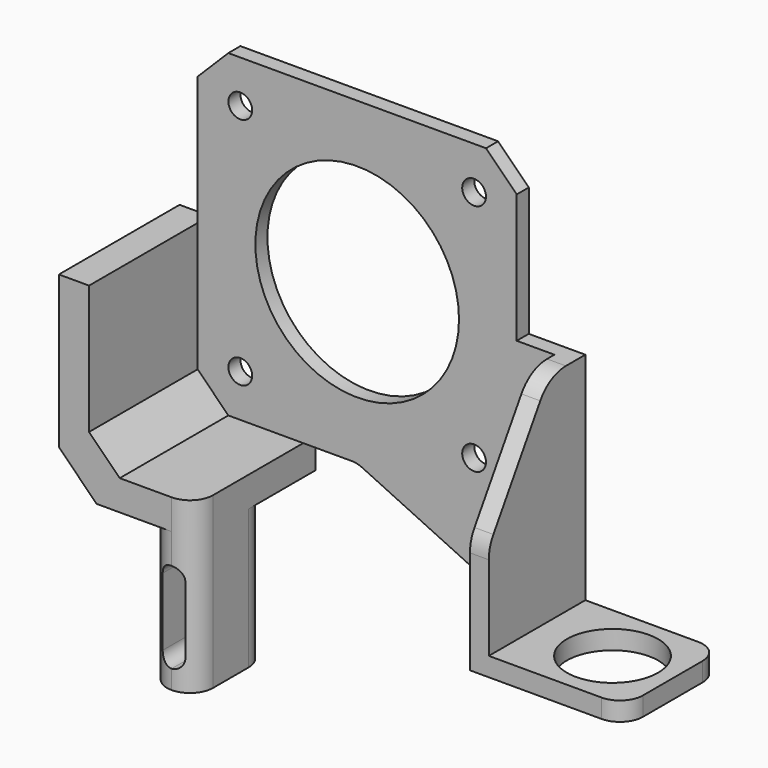
from build123d import *

# Parameters (mm, degrees)
F0_R         = 1.575
F0_R_2       = 13.5
F0_W         = 5
F0_H         = 21.15
F1_DEPTH     = 2
F2_DEPTH     = 20
F3_DEPTH     = 16
F4_R         = 6.05
F5_DEPTH     = 2.5
F6_W         = 6.1
F6_H         = 12
F7_DEPTH     = 18.5
F8_W         = 3
F8_H         = 12
F9_DEPTH     = 12
F10_T1_DEPTH = 2
F10_T3_DEPTH = 26.125
F10_T5_DEPTH = 37.75
F10_T7_DEPTH = 17.75
F10_T9_DEPTH = 5.4173756904
F11_R        = 1.49999
F12_SIZE     = 5
F13_SIZE2    = 16
F13_SIZE     = 10
F14_R        = 5


# Not quite as in the source:
# - a fillet or chamfer that OpenCascade refuses, or shapes differently, is made with other operations: its cross-section is extruded or revolved along the edge and cut away or added
# - a fillet or chamfer is up to 0.001 mm smaller than in the source, because OpenCascade refuses the exact size
# - a feature names something its author has since deleted; it is built from what else it names


with BuildPart() as f1:
    # F0 (on Front) → F1 (new body)
    with BuildSketch(Plane.XZ):
        Polygon((-21.15, -17.0841360082), (-21.15, 0), (-25.15, 0), (-25.15, -25.15), (-7.15, -25.15), (-7.15, -21.15), (-17.0841360082, -21.15), (-21.15, -21.15), align=None)
        Polygon((21.15, 17.0841360082), (17.0841360082, 21.15), (-17.0841360082, 21.15), (-21.15, 17.0841360082), (-21.15, 0), (-21.15, -17.0841360082), (-17.0841360082, -21.15), (-7.15, -21.15), (0, -21.15), (21.15, -21.15), (21.15, 0), align=None)
        with Locations((-15.5, -15.5)):
            Circle(F0_R, mode=Mode.SUBTRACT)
        with Locations((15.5, -15.5)):
            Circle(F0_R, mode=Mode.SUBTRACT)
        Circle(F0_R_2, mode=Mode.SUBTRACT)
        with Locations((-15.5, 15.5)):
            Circle(F0_R, mode=Mode.SUBTRACT)
        with Locations((15.5, 15.5)):
            Circle(F0_R, mode=Mode.SUBTRACT)
        Polygon((-17.0841360082, -21.15), (-21.15, -17.0841360082), (-21.15, -21.15), align=None)
        Polygon((26.15, -21.15), (21.15, -21.15), (0, -21.15), (21.1919918656, -31.15), (26.15, -31.15), align=None)
        Polygon((28.65, 0), (26.15, 0), (26.15, -21.15), (26.15, -31.15), (46.65, -31.15), (46.65, -28.65), (28.65, -28.65), align=None)
        with Locations((23.65, -10.575)):
            Rectangle(F0_W, F0_H)
    extrude(amount=F1_DEPTH)

    # F0 (on Front) → F2 (join)
    with BuildSketch(Plane.XZ):
        Polygon((-21.15, -17.0841360082), (-21.15, 0), (-25.15, 0), (-25.15, -25.15), (-7.15, -25.15), (-7.15, -21.15), (-17.0841360082, -21.15), (-21.15, -21.15), align=None)
        Polygon((-17.0841360082, -21.15), (-21.15, -17.0841360082), (-21.15, -21.15), align=None)
    extrude(amount=F2_DEPTH)

    # F0 (on Front) → F3 (join)
    with BuildSketch(Plane.XZ):
        Polygon((28.65, 0), (26.15, 0), (26.15, -21.15), (26.15, -31.15), (46.65, -31.15), (46.65, -28.65), (28.65, -28.65), align=None)
    extrude(amount=F3_DEPTH)

    # F4 (on face) → F5 (cut, through all)
    with BuildSketch(Plane.XY.offset(-28.65)):
        with Locations((38.65, -8)):
            Circle(F4_R)
    extrude(amount=-F5_DEPTH, mode=Mode.SUBTRACT)

    # F6 (on face) → F7 (join)
    with BuildSketch(Plane(origin=(0, 0, -25.15), x_dir=(1, 0, 0), z_dir=(0, 0, -1))):
        with Locations((-10.2, 14)):
            Rectangle(F6_W, F6_H)
    extrude(amount=F7_DEPTH)

    # F8 (on face) → F9 (cut, through all)
    with BuildSketch(Plane.XZ.offset(20)):
        with Locations((-10.2, -35.15)):
            Rectangle(F8_W, F8_H)
    extrude(amount=-F9_DEPTH, mode=Mode.SUBTRACT)

    # F10: fillet of radius 3.05 on 8 edges, made by hand

    # F10_s2 → F10_t1 (join)
    with BuildSketch(Plane.XZ):
        with BuildLine():
            ThreePointArc((-0.6834751381, -21.15), (-0.0165404304, -21.2238114818), (0.6181139894, -21.4416733799))
            Line((0.6181139894, -21.4416733799), (0, -21.15))
            Line((0, -21.15), (-0.6834751381, -21.15))
        make_face()
    extrude(amount=F10_T1_DEPTH)

    # F10_s4 → F10_t3 (cut)
    with BuildSketch(Plane.XY.offset(-51.275)):
        with BuildLine():
            ThreePointArc((-13.25, -11.05), (-12.3566756826, -8.8933243174), (-10.2, -8))
            Line((-10.2, -8), (-13.25, -8))
            Line((-13.25, -8), (-13.25, -11.05))
        make_face()
        with BuildLine():
            ThreePointArc((-7.15, -11.05), (-8.0433243174, -8.8933243174), (-10.2, -8))
            Line((-10.2, -8), (-7.15, -8))
            Line((-7.15, -8), (-7.15, -11.05))
        make_face()
        with BuildLine():
            ThreePointArc((-10.2, -20), (-12.3566756826, -19.1066756826), (-13.25, -16.95))
            Line((-13.25, -16.95), (-13.25, -20))
            Line((-13.25, -20), (-10.2, -20))
        make_face()
    extrude(amount=F10_T3_DEPTH, mode=Mode.SUBTRACT)

    # F10_s6 → F10_t5 (cut)
    with BuildSketch(Plane.XY.offset(-51.275)):
        with BuildLine():
            ThreePointArc((-10.2, -20), (-8.0433243174, -19.1066756826), (-7.15, -16.95))
            Line((-7.15, -16.95), (-7.15, -20))
            Line((-7.15, -20), (-10.2, -20))
        make_face()
    extrude(amount=F10_T5_DEPTH, mode=Mode.SUBTRACT)

    # F10_s8 → F10_t7 (cut)
    with BuildSketch(Plane.XY.offset(-38.775)):
        with BuildLine():
            ThreePointArc((46.65, -12.95), (45.7566756826, -15.1066756826), (43.6, -16))
            Line((43.6, -16), (46.65, -16))
            Line((46.65, -16), (46.65, -12.95))
        make_face()
        with BuildLine():
            ThreePointArc((43.6, 0), (45.7566756826, -0.8933243174), (46.65, -3.05))
            Line((46.65, -3.05), (46.65, 0))
            Line((46.65, 0), (43.6, 0))
        make_face()
    extrude(amount=F10_T7_DEPTH, mode=Mode.SUBTRACT)

    # F10_s10 → F10_t9 (cut)
    with BuildSketch(Plane.XZ.offset(-1.7086878452)):
        with BuildLine():
            ThreePointArc((20.5738778763, -30.8583266201), (21.208532296, -31.0761885182), (21.8754670037, -31.15))
            Line((21.8754670037, -31.15), (21.1919918656, -31.15))
            Line((21.1919918656, -31.15), (20.5738778763, -30.8583266201))
        make_face()
    extrude(amount=F10_T9_DEPTH, mode=Mode.SUBTRACT)

    # F11 (radius 1.5 in the source; OpenCascade refuses exactly that, so slightly less here)
    f11_edges = [f1.edges().sort_by_distance(p)[0] for p in [
        (-11.7, -14, -29.15),
        (-8.7, -14, -29.15),
        (-11.7, -14, -41.15),
        (-8.7, -14, -41.15),
    ]]
    fillet(f11_edges, radius=F11_R)

    # F12
    f12_edges = [f1.edges().sort_by_distance(p)[0] for p in [
        (-25.15, -10, -25.15),
    ]]
    chamfer(f12_edges, length=F12_SIZE)

    # F13
    f13_edges = [f1.edges().sort_by_distance(p)[0] for p in [
        (27.4, -16, 0),
    ]]
    f13_side = f1.faces().sort_by_distance((26.65, -6.6, 0))[0]
    chamfer(f13_edges, length=F13_SIZE, length2=F13_SIZE2, reference=f13_side)

    # F14
    f14_edges = [f1.edges().sort_by_distance(p)[0] for p in [
        (27.4, -16, -16),
        (27.4, -6, 0),
    ]]
    fillet(f14_edges, radius=F14_R)


solid = f1.part
